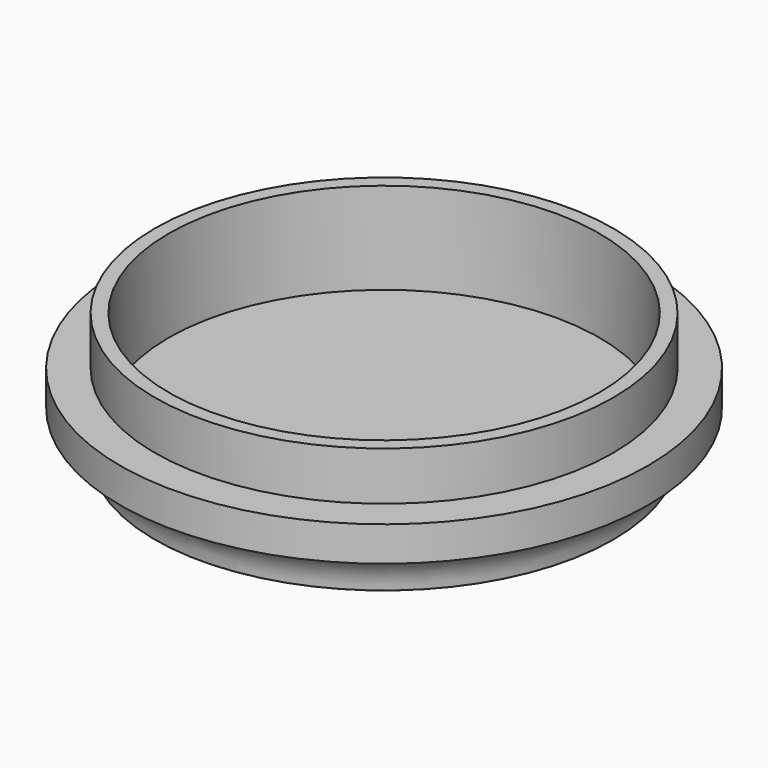
from build123d import *

# Parameters (mm, degrees)
F0_R     = 16.5
F1_DEPTH = 9
F4_R     = 19
F5_DEPTH = 2.5
F2_R     = 15.5
F6_DEPTH = 6.6


# Not quite as in the source:
# - a fillet or chamfer that OpenCascade refuses, or shapes differently, is made with other operations: its cross-section is extruded or revolved along the edge and cut away or added


with BuildPart() as f1:
    # F0 (on Top) → F1 (new body)
    with BuildSketch(Plane.XY):
        Circle(F0_R)
    extrude(amount=F1_DEPTH)

    # F4 (on offset) → F5 (join)
    with BuildSketch(Plane.XY.offset(5.5)):
        Circle(F4_R)
    extrude(amount=-F5_DEPTH)

    # F2 (on face) → F6 (cut)
    with BuildSketch(Plane.XY.offset(9)):
        Circle(F2_R)
    extrude(amount=-F6_DEPTH, mode=Mode.SUBTRACT)

    # F7: fillet of radius 3 on 1 edges, made by hand

    # F7_s1 → F7_t2 (revolve)
    with BuildSketch(Plane.XZ):
        with BuildLine():
            ThreePointArc((16.5, 0.0419601084), (17.2087121525, 1.9784517816), (19, 3))
            Line((19, 3), (16.5, 3))
            Line((16.5, 3), (16.5, 0.0419601084))
        make_face()
    revolve(axis=Axis((0, 0, 3), (0, 0, -1)))


solid = f1.part
